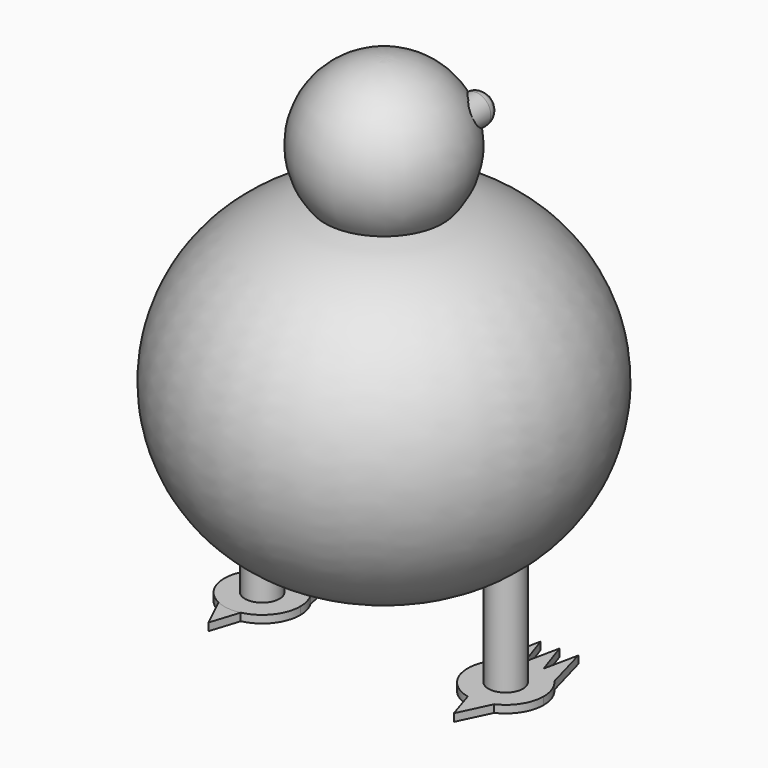
from build123d import *

# Parameters (mm, degrees)
F0_R           = 2.8916080187
F1_DEPTH       = 25.4
F4_DEPTH       = 1.27
F5_DEPTH       = 1.27
F6_DEPTH       = 1.27
F14_R          = 2.54
F15_DEPTH      = 0.762
F15_DEPTH_BACK = 5.6642
F16_R          = 2.2225
F16_2_R        = 2.2225


# Not quite as in the source:
# - the program builds the solid bodies; features that only make, move or delete a surface that nothing else refers to are left out


with BuildPart() as f1:
    # F0 (on Top) → F1 (new body)
    with BuildSketch(Plane.XY):
        with Locations((-20.32, 0)):
            Circle(F0_R)
    extrude(amount=F1_DEPTH)

    # F0 (on Top) → F4 (join)
    with BuildSketch(Plane.XY):
        with BuildLine():
            ThreePointArc((-18.9462788097, -6.199628222), (-15.3679484273, -3.974881787), (-13.97, 0))
            ThreePointArc((-13.97, 0), (-14.1967687766, 1.6818262053), (-14.8608785464, 3.2435309394))
            ThreePointArc((-14.8608785464, 3.2435309394), (-16.4582285071, 5.0407559886), (-18.6092892941, 6.1152243524))
            ThreePointArc((-18.6092892941, 6.1152243524), (-20.1637925957, 6.3480783901), (-21.7278672749, 6.1919633184))
            Line((-21.7278672749, 6.1919633184), (-21.7538577959, 6.1152243524))
            Line((-21.7538577959, 6.1152243524), (-21.7680442692, 6.1826909833))
            ThreePointArc((-21.7680442692, 6.1826909833), (-23.5685523861, 5.4561348402), (-25.0653563388, 4.2194896869))
            ThreePointArc((-25.0653563388, 4.2194896869), (-26.5392399855, -1.2820117015), (-23.0098377174, -5.7521537753))
            ThreePointArc((-23.0098377174, -5.7521537753), (-21.0150532522, -6.3118460831), (-18.9462788097, -6.199628222))
        make_face()
        with Locations((-20.32, 0)):
            Circle(F0_R, mode=Mode.SUBTRACT)
    extrude(amount=F4_DEPTH)

    # F0 (on Top) → F5 (join)
    with BuildSketch(Plane.XY):
        with BuildLine():
            Line((-22.9583520449, 11.8434393375), (-25.0653563388, 4.2194896869))
            ThreePointArc((-25.0653563388, 4.2194896869), (-23.5685523861, 5.4561348402), (-21.7680442692, 6.1826909833))
            Line((-21.7680442692, 6.1826909833), (-22.9583520449, 11.8434393375))
        make_face()
    extrude(amount=F5_DEPTH)


with BuildPart() as f1b:
    # F0 (on Top) → F1, piece 2 (new body)
    with BuildSketch(Plane.XY):
        with Locations((20.32, 0)):
            Circle(F0_R)
    extrude(amount=F1_DEPTH)


with BuildPart() as f3:
    # F2 (on Front) → F3 (revolve)
    with BuildSketch(Plane.XZ):
        with BuildLine():
            Line((0, 12.6862702891), (0, 65.1613026857))
            ThreePointArc((0, 65.1613026857), (-32.1425145903, 38.9237864874), (0, 12.6862702891))
        make_face()
    revolve(axis=Axis((0, 0, 38.9237864874), (0, 0, -1)))

    # F7 (on Front) → F8 (revolve)
    with BuildSketch(Plane.XZ):
        with BuildLine():
            ThreePointArc((0, 86.3951636095), (-13.0087475703, 73.6951636095), (0, 60.9951636095))
            Line((0, 60.9951636095), (0, 86.3951636095))
        make_face()
    revolve(axis=Axis((0, 0, 73.6951636095), (0, 0, 1)))


with BuildPart() as f6:
    # F0 (on Top) → F6 (new body)
    with BuildSketch(Plane.XY):
        with BuildLine():
            ThreePointArc((-21.7278672749, 6.1919633184), (-20.1637925957, 6.3480783901), (-18.6092892941, 6.1152243524))
            Line((-18.6092892941, 6.1152243524), (-19.813783543, 11.8434393375))
            Line((-19.813783543, 11.8434393375), (-21.7278672749, 6.1919633184))
        make_face()
    extrude(amount=F6_DEPTH)


with BuildPart() as f6b:
    # F0 (on Top) → F6, piece 2 (new body)
    with BuildSketch(Plane.XY):
        with BuildLine():
            ThreePointArc((-18.6092892941, 6.1152243524), (-16.4582285071, 5.0407559886), (-14.8608785464, 3.2435309394))
            Line((-14.8608785464, 3.2435309394), (-16.6692150412, 11.8434393375))
            Line((-16.6692150412, 11.8434393375), (-18.6092892941, 6.1152243524))
        make_face()
    extrude(amount=F6_DEPTH)


with BuildPart() as f6c:
    # F0 (on Top) → F6, piece 3 (new body)
    with BuildSketch(Plane.XY):
        with BuildLine():
            Line((-20.4855929921, -11.0407966603), (-18.9462788097, -6.199628222))
            ThreePointArc((-18.9462788097, -6.199628222), (-21.0150532522, -6.3118460831), (-23.0098377174, -5.7521537753))
            Line((-23.0098377174, -5.7521537753), (-20.4855929921, -11.0407966603))
        make_face()
    extrude(amount=F6_DEPTH)


with BuildPart() as f6d:
    # F0 (on Top) → F6, piece 4 (new body)
    with BuildSketch(Plane.XY):
        with BuildLine():
            ThreePointArc((23.0098377174, -5.7521537753), (21.0150532522, -6.3118460831), (18.9462788097, -6.199628222))
            Line((18.9462788097, -6.199628222), (20.4855929921, -11.0407966603))
            Line((20.4855929921, -11.0407966603), (23.0098377174, -5.7521537753))
        make_face()
        with BuildLine():
            Line((16.6692150412, 11.8434393375), (14.8608785464, 3.2435309394))
            ThreePointArc((14.8608785464, 3.2435309394), (16.4582285071, 5.0407559886), (18.6092892941, 6.1152243524))
            Line((18.6092892941, 6.1152243524), (16.6692150412, 11.8434393375))
        make_face()
        with BuildLine():
            Line((19.813783543, 11.8434393375), (18.6092892941, 6.1152243524))
            ThreePointArc((18.6092892941, 6.1152243524), (20.1637925957, 6.3480783901), (21.7278672749, 6.1919633184))
            Line((21.7278672749, 6.1919633184), (19.813783543, 11.8434393375))
        make_face()
        with BuildLine():
            ThreePointArc((14.8608785464, 3.2435309394), (14.4920287933, -2.5213590807), (18.9462788097, -6.199628222))
            ThreePointArc((18.9462788097, -6.199628222), (21.0150532522, -6.3118460831), (23.0098377174, -5.7521537753))
            ThreePointArc((23.0098377174, -5.7521537753), (25.677376667, -3.4089610217), (26.67, 0))
            ThreePointArc((26.67, 0), (26.2552974968, 2.257153877), (25.0653563388, 4.2194896869))
            ThreePointArc((25.0653563388, 4.2194896869), (23.5685523861, 5.4561348402), (21.7680442692, 6.1826909833))
            Line((21.7680442692, 6.1826909833), (21.7538577959, 6.1152243524))
            Line((21.7538577959, 6.1152243524), (21.7278672749, 6.1919633184))
            ThreePointArc((21.7278672749, 6.1919633184), (20.1637925957, 6.3480783901), (18.6092892941, 6.1152243524))
            ThreePointArc((18.6092892941, 6.1152243524), (16.4582285071, 5.0407559886), (14.8608785464, 3.2435309394))
        make_face()
        with Locations((20.32, 0)):
            Circle(F0_R, mode=Mode.SUBTRACT)
        with BuildLine():
            ThreePointArc((21.7680442692, 6.1826909833), (23.5685523861, 5.4561348402), (25.0653563388, 4.2194896869))
            Line((25.0653563388, 4.2194896869), (22.9583520449, 11.8434393375))
            Line((22.9583520449, 11.8434393375), (21.7680442692, 6.1826909833))
        make_face()
    extrude(amount=F6_DEPTH)


with BuildPart() as f15:
    # F14 (on offset) → F15 (new body, two sides)
    with BuildSketch(Plane.XZ.offset(-10.16)) as f15_sk:
        with Locations((8.3199816652, 78.0233695126)):
            Circle(F14_R)
    extrude(amount=-F15_DEPTH)
    extrude(f15_sk.sketch, amount=F15_DEPTH_BACK)

    # F16
    f16_edges = [f15.edges().sort_by_distance(p)[0] for p in [
        (5.779982, 10.922, 78.02337),
    ]]
    fillet(f16_edges, radius=F16_R)


with BuildPart() as f15b:
    # F14 (on offset) → F15, piece 2 (new body, two sides)
    with BuildSketch(Plane.XZ.offset(-10.16)) as f15_2_sk:
        with Locations((-8.3199816652, 78.0233695126)):
            Circle(F14_R)
    extrude(amount=-F15_DEPTH)
    extrude(f15_2_sk.sketch, amount=F15_DEPTH_BACK)

    # F16#2
    f16_2_edges = [f15b.edges().sort_by_distance(p)[0] for p in [
        (-10.859982, 10.922, 78.02337),
    ]]
    fillet(f16_2_edges, radius=F16_2_R)


solid = Compound([f1.part, f1b.part, f3.part, f6.part, f6b.part, f6c.part, f6d.part, f15.part, f15b.part])
